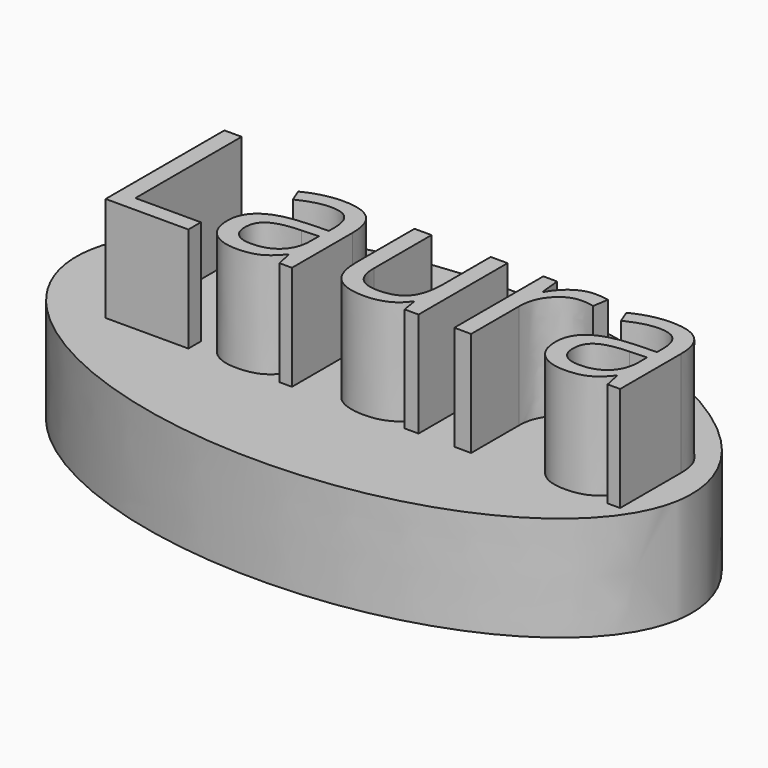
from build123d import *

# Parameters (mm, degrees)
F1_DEPTH     = 25.4
F2_TEXT_SIZE = 50.39605469
F3_DEPTH     = 25.4


# Not quite as in the source:
# - Text() gives the source's letters only with a copy of the font that has no kerning and outlines rounded to 1/6400 em; it was checked with that copy


with BuildPart() as f1:
    # F0 (on Top) → F1 (new body)
    with BuildSketch(Plane.XY):
        with BuildLine():
            add(Edge.make_bspline(
                [(75.8589357138, -2.289499389), (78.0649010029, 70.8016662408), (-36.8264852123, 37.6903325094), (-151.7178714275, 4.578998778), (-39.0324505014, -35.4008331204), (73.6529704247, -75.3806650188), (75.8589357138, -2.289499389)],
                knots=[0, 0, 0, 2.0943951024, 2.0943951024, 4.1887902048, 4.1887902048, 6.2831853072, 6.2831853072, 6.2831853072], degree=2, weights=[1, 0.5, 1, 0.5, 1, 0.5, 1]))
        make_face()
    extrude(amount=F1_DEPTH)

    # F2 (on face) → F3 (join)
    with BuildSketch(Plane.XY.offset(25.4)):
        with Locations((-60.7563869765, -14.5686822489)):
            Text('Laura', F2_TEXT_SIZE, font='Open Sans', text_align=(TextAlign.LEFT, TextAlign.BOTTOM))
    extrude(amount=F3_DEPTH)


solid = f1.part
